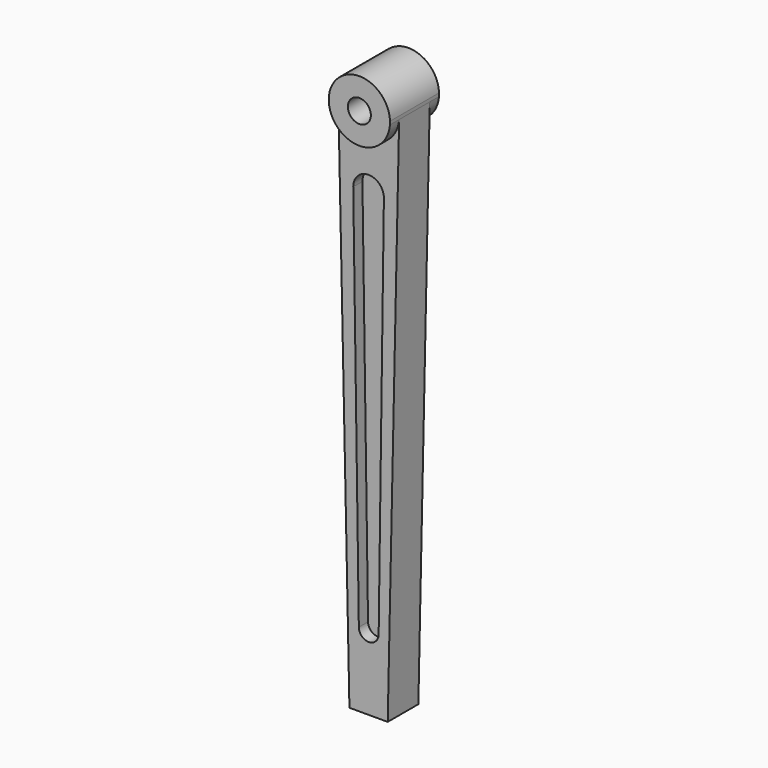
from build123d import *

# Parameters (mm, degrees)
F1_DEPTH = 2.5
F0_R     = 1.5
F2_DEPTH = 4
F3_DEPTH = 1


# Not quite as in the source:
# - a feature names something its author has since deleted; it is built from what else it names


with BuildPart() as f1:
    # F0 (on Front) → F1 (new body, symmetric)
    with BuildSketch(Plane.XZ):
        with BuildLine():
            Line((-3.9449856715, 23.9478669513), (-2.5, -45.3910091387))
            Line((-2.5, -45.3910091387), (2.5, -45.3910091387))
            Line((2.5, -45.3910091387), (3.9887932138, 24.3097798378))
            ThreePointArc((3.9887932138, 24.3097798378), (0.1822772875, 20.6131485868), (-3.9449856715, 23.9478669513))
        make_face()
        with BuildLine():
            ThreePointArc((-1.9997903124, 14.6349845216), (-0.0009328581, 16.6639447346), (1.9998164582, 14.6368500546))
            Line((1.9998164582, 14.6368500546), (1.3173793796, -35.7323714856))
            ThreePointArc((1.3173793796, -35.7323714856), (0.0241016903, -37.0088409461), (-1.270366201, -35.7335784854))
            Line((-1.270366201, -35.7335784854), (-1.9997903124, 14.6349845216))
        make_face(mode=Mode.SUBTRACT)
    extrude(amount=F1_DEPTH, both=True)

    # F0 (on Front) → F2 (join, symmetric)
    with BuildSketch(Plane.XZ):
        with BuildLine():
            Line((-3.9691037619, 25.1051941963), (-3.9449856715, 23.9478669513))
            ThreePointArc((-3.9449856715, 23.9478669513), (0.1822772875, 20.6131485868), (3.9887932138, 24.3097798378))
            Line((3.9887932138, 24.3097798378), (3.9979316153, 24.7376121165))
            ThreePointArc((3.9979316153, 24.7376121165), (0.184355384, 28.6047426804), (-3.9691037619, 25.1051941963))
        make_face()
        with Locations((0, 24.6089933023)):
            Circle(F0_R, mode=Mode.SUBTRACT)
    extrude(amount=F2_DEPTH, both=True)

    # F0 (on Front) → F3 (join, symmetric)
    with BuildSketch(Plane.XZ):
        with BuildLine():
            Line((1.3173793796, -35.7323714856), (1.9998164582, 14.6368500546))
            ThreePointArc((1.9998164582, 14.6368500546), (-0.0009328581, 16.6639447346), (-1.9997903124, 14.6349845216))
            Line((-1.9997903124, 14.6349845216), (-1.270366201, -35.7335784854))
            ThreePointArc((-1.270366201, -35.7335784854), (0.0241016903, -37.0088409461), (1.3173793796, -35.7323714856))
        make_face()
    extrude(amount=F3_DEPTH, both=True)


solid = f1.part
